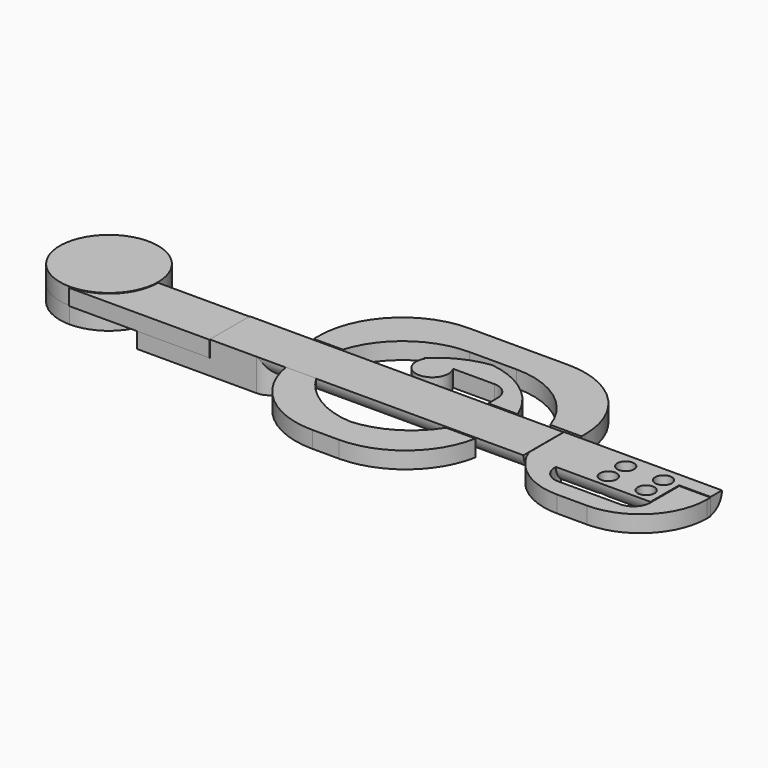
from build123d import *

# Parameters (mm, degrees)
F0_W           = 74.9647691846
F0_H           = 4.8156478442
F0_W_2         = 21.8120515347
F1_DEPTH       = 7.5
F2_T1_DEPTH    = 87.4562698657
F2_T3_DEPTH    = 17.3156478442
F2_T9_DEPTH    = 87.4562698657
F2_T13_DEPTH   = 17.3156478442
F2_T21_DEPTH   = 87.4562698657
F2_T25_DEPTH   = 17.3156478442
F4_DEPTH       = 4.8
F5_DEPTH       = 5
F6_W           = 9.4357505441
F6_H           = 4.2491005734
F7_DEPTH       = 5
F8_R           = 4.99999
F9_W           = 9.3480274081
F9_H           = 5.3821951151
F9_W_2         = 9.3480348587
F9_H_2         = 4.8156473786
F9_H_3         = 5.5238311179
F9_W_3         = 28.6106020212
F10_DEPTH      = 5
F11_T1_DEPTH   = 98.1931302685
F11_T3_DEPTH   = 105
F13_D          = 5
F14_D          = 5
F15_D          = 5
F16_D          = 5
F17_W          = 9.3480274081
F17_H          = 16.9964022934
F17_W_2        = 61.7535989732
F17_H_2        = 9.3480236828
F18_DEPTH      = 5
F17_W_3        = 9.0647486504
F17_H_3        = 12.1807572432
F17_H_4        = 8.7814740837
F17_W_4        = 39.374999702
F17_W_5        = 8.7814815342
F17_H_5        = 11.6142109036
F17_H_6        = 8.5145081393
F17_W_6        = 26.0611474514
F17_H_7        = 7.3767574504
F19_T1_DEPTH   = 5
F19_T3_DEPTH   = 5
F19_T5_DEPTH   = 130
F19_T7_DEPTH   = 130
F19_2_T1_DEPTH = 5
F19_2_T3_DEPTH = 127.8617396979
F19_2_T5_DEPTH = 128.3588691726
F19_3_T1_DEPTH = 121.4077915609
F19_3_T3_DEPTH = 93.6596472526
F20_R          = 4.8994331179
F21_DEPTH      = 5
F22_R          = 5
F22_2_R        = 5


# Not quite as in the source:
# - a fillet or chamfer that OpenCascade refuses, or shapes differently, is made with other operations: its cross-section is extruded or revolved along the edge and cut away or added
# - a fillet or chamfer is up to 0.001 mm smaller than in the source, because OpenCascade refuses the exact size


with BuildPart() as f1:
    # F0 (on Front) → F1 (new body, symmetric)
    with BuildSketch(Plane.XZ):
        with Locations((37.4823845923, 2.4078239221)):
            Rectangle(F0_W, F0_H)
        Polygon((0, -4.8156478442), (0, 0), (0, 4.8156478442), (-19.0819986165, 4.8156478442), (-19.0819986165, 0), (-19.0819986165, -4.8156478442), align=None)
        with Locations((-29.9880243838, -2.4078239221)):
            Rectangle(F0_W_2, F0_H)
    extrude(amount=F1_DEPTH, both=True)

    # F2: fillet of radius 5 on 4 edges, made by hand

    # F2_s2 → F2_t1 (cut)
    with BuildSketch(Plane.YZ):
        with BuildLine():
            ThreePointArc((-2.5033997275, 0), (-5.9731431778, 1.3998777258), (-7.5, 4.8156478442))
            Line((-7.5, 4.8156478442), (-7.5, 0))
            Line((-7.5, 0), (-2.5033997275, 0))
        make_face()
        with BuildLine():
            ThreePointArc((2.5033997275, 0), (5.9731431778, 1.3998777258), (7.5, 4.8156478442))
            Line((7.5, 4.8156478442), (7.5, 0))
            Line((7.5, 0), (2.5033997275, 0))
        make_face()
    extrude(amount=F2_T1_DEPTH, mode=Mode.SUBTRACT)

    # F2_s4 → F2_t3 (cut)
    with BuildSketch(Plane.XY.offset(-17.3156478442)):
        with BuildLine():
            ThreePointArc((0, -2.5), (-1.4644660941, -6.0355339059), (-5, -7.5))
            Line((-5, -7.5), (0, -7.5))
            Line((0, -7.5), (0, -2.5))
        make_face()
        with BuildLine():
            ThreePointArc((0, 2.5), (-1.4644660941, 6.0355339059), (-5, 7.5))
            Line((-5, 7.5), (0, 7.5))
            Line((0, 7.5), (0, 2.5))
        make_face()
    extrude(amount=F2_T3_DEPTH, mode=Mode.SUBTRACT)


with BuildPart() as f2_tool7:
    # F2_s8 → F2_t9 (new body)
    with BuildSketch(Plane.YZ.offset(-12.4915006811)):
        with BuildLine():
            ThreePointArc((-2.5033997275, 0), (-5.9731431778, 1.3998777258), (-7.5, 4.8156478442))
            Line((-7.5, 4.8156478442), (-7.5, 0))
            Line((-7.5, 0), (-2.5033997275, 0))
        make_face()
    extrude(amount=F2_T9_DEPTH)

    split(bisect_by=Plane.YZ, keep=Keep.BOTTOM)


with BuildPart() as f2_tool11:
    # F2_s12 → F2_t13 (new body)
    with BuildSketch(Plane.XY.offset(-4.8156478442)):
        with BuildLine():
            ThreePointArc((0, -2.5), (-1.4644660941, -6.0355339059), (-5, -7.5))
            Line((-5, -7.5), (0, -7.5))
            Line((0, -7.5), (0, -2.5))
        make_face()
    extrude(amount=F2_T13_DEPTH)

    split(bisect_by=Plane.XY, keep=Keep.TOP)

    split(bisect_by=Plane.XY.offset(4.8156478442), keep=Keep.BOTTOM)


with BuildPart() as f2_tool7_1:
    add(f2_tool7.part)

    # F2_t16: intersect F2_tool11
    add(f2_tool11.part, mode=Mode.INTERSECT)


with BuildPart() as f1_1:
    add(f1.part)

    # F2_t5: cut F2_tool7
    add(f2_tool7_1.part, mode=Mode.SUBTRACT)


with BuildPart() as f2_tool19:
    # F2_s20 → F2_t21 (new body)
    with BuildSketch(Plane.YZ.offset(-12.4915006811)):
        with BuildLine():
            ThreePointArc((2.5033997275, 0), (5.9731431778, 1.3998777258), (7.5, 4.8156478442))
            Line((7.5, 4.8156478442), (7.5, 0))
            Line((7.5, 0), (2.5033997275, 0))
        make_face()
    extrude(amount=F2_T21_DEPTH)

    split(bisect_by=Plane.YZ, keep=Keep.BOTTOM)


with BuildPart() as f2_tool23:
    # F2_s24 → F2_t25 (new body)
    with BuildSketch(Plane.XY.offset(-4.8156478442)):
        with BuildLine():
            ThreePointArc((0, 2.5), (-1.4644660941, 6.0355339059), (-5, 7.5))
            Line((-5, 7.5), (0, 7.5))
            Line((0, 7.5), (0, 2.5))
        make_face()
    extrude(amount=F2_T25_DEPTH)

    split(bisect_by=Plane.XY, keep=Keep.TOP)

    split(bisect_by=Plane.XY.offset(4.8156478442), keep=Keep.BOTTOM)


with BuildPart() as f2_tool19_1:
    add(f2_tool19.part)

    # F2_t28: intersect F2_tool23
    add(f2_tool23.part, mode=Mode.INTERSECT)


with BuildPart() as f1_2:
    add(f1_1.part)

    # F2_t17: cut F2_tool19
    add(f2_tool19_1.part, mode=Mode.SUBTRACT)

    # F3 (on Top) → F4 (join)
    with BuildSketch(Plane.XY):
        with BuildLine():
            Line((-61.1870549619, -7.6483818702), (-18.97931844, -7.6483818702))
            Line((-18.97931844, -7.6483818702), (-18.97931844, 7.3651091661))
            Line((-18.97931844, 7.3651091661), (-46.4570610243, 7.3651091661))
            ThreePointArc((-46.4570610243, 7.3651091661), (-50.7713763618, -3.050569434), (-61.1870549619, -7.3648847715))
            Line((-61.1870549619, -7.3648847715), (-61.1870549619, -7.6483818702))
        make_face()
    extrude(amount=F4_DEPTH)

    # F3 (on Top) → F5 (join, symmetric)
    with BuildSketch(Plane.XY):
        with BuildLine():
            ThreePointArc((-46.4570610243, 7.3651091661), (-71.602733562, 17.7807877663), (-61.1870549619, -7.3648847715))
            Line((-61.1870549619, -7.3648847715), (-61.1870549619, 7.3651091661))
            Line((-61.1870549619, 7.3651091661), (-46.4570610243, 7.3651091661))
        make_face()
        with BuildLine():
            Line((-61.1870549619, 7.3651091661), (-61.1870549619, -7.3648847715))
            ThreePointArc((-61.1870549619, -7.3648847715), (-50.7713763618, -3.050569434), (-46.4570610243, 7.3651091661))
            Line((-46.4570610243, 7.3651091661), (-61.1870549619, 7.3651091661))
        make_face()
    extrude(amount=F5_DEPTH, both=True)


with BuildPart() as f7:
    # F6 (on Top) → F7 (new body)
    with BuildSketch(Plane.XY):
        Polygon((75.2632021904, 7.365108002), (75.2632021904, -7.6483818702), (113.1341084838, -7.6483818702), (113.1341084838, 3.1160074286), (113.1341084838, 7.365108002), align=None)
        with Locations((117.8519837558, 5.2405577153)):
            Rectangle(F6_W, F6_H)
    extrude(amount=F7_DEPTH)

    # F8 (radius 5 in the source; OpenCascade refuses exactly that, so slightly less here)
    f8_edges = [f7.edges().sort_by_distance(p)[0] for p in [
        (94.198655, -7.648382, 0),
        (98.916531, 7.365108, 0),
    ]]
    fillet(f8_edges, radius=F8_R)

    # F9 (on Top) → F10 (join)
    with BuildSketch(Plane.XY):
        with Locations((80.1227204502, -15.7216731459)):
            Rectangle(F9_W, F9_H)
        Polygon((75.4487067461, -13.0305755883), (84.7967341542, -13.0305755883), (84.7967341542, -5.665468052), (75.1654356718, -5.665468052), (75.1654356718, -18.4127707034), (75.4487067461, -18.4127707034), align=None)
        with Locations((118.0813536048, -15.7216731459)):
            Rectangle(F9_W_2, F9_H)
        with Locations((118.0813536048, -10.6227518991)):
            Rectangle(F9_W_2, F9_H_2)
        with Locations((118.0813536048, -5.4530126508)):
            Rectangle(F9_W_2, F9_H_3)
        with Locations((118.0813536048, 0.0708184671)):
            Rectangle(F9_W_2, F9_H_3)
        with Locations((99.1020351648, -15.7216731459)):
            Rectangle(F9_W_3, F9_H)
    extrude(amount=F10_DEPTH)

    # F11: fillet of radius 20 on 2 edges, made by hand

    # F11_s2 → F11_t1 (cut)
    with BuildSketch(Plane.XY.offset(-46.5965651343)):
        with BuildLine():
            ThreePointArc((75.1654356718, -5.665468052), (82.5136664041, -14.9211617058), (93.8040617255, -18.4127707034))
            Line((93.8040617255, -18.4127707034), (75.1654356718, -18.4127707034))
            Line((75.1654356718, -18.4127707034), (75.1654356718, -5.665468052))
        make_face()
    extrude(amount=F11_T1_DEPTH, mode=Mode.SUBTRACT)

    # F11_s4 → F11_t3 (cut)
    with BuildSketch(Plane.XY.offset(-50)):
        with BuildLine():
            ThreePointArc((102.7553710341, -18.4127707034), (116.8975066579, -12.5549063272), (122.7553710341, 1.5872292966))
            Line((122.7553710341, 1.5872292966), (122.7553710341, -18.4127707034))
            Line((122.7553710341, -18.4127707034), (102.7553710341, -18.4127707034))
        make_face()
    extrude(amount=F11_T3_DEPTH, mode=Mode.SUBTRACT)

    # F13 (through all)
    with Locations(Plane(origin=(0, 0, 0), x_dir=(1, 0, 0), z_dir=(0, 0, -1))):
        with Locations((97.3535180092, -2.832734026)):
            Hole(F13_D / 2)

    # F14 (through all)
    with Locations(Plane(origin=(0, 0, 0), x_dir=(1, 0, 0), z_dir=(0, 0, -1))):
        with Locations((97.3535180092, 3.682554001)):
            Hole(F14_D / 2)

    # F15 (through all)
    with Locations(Plane(origin=(0, 0, 0), x_dir=(1, 0, 0), z_dir=(0, 0, -1))):
        with Locations((108.684450388, -2.832734026)):
            Hole(F15_D / 2)

    # F16 (through all)
    with Locations(Plane(origin=(0, 0, 0), x_dir=(1, 0, 0), z_dir=(0, 0, -1))):
        with Locations((108.684450388, 3.682554001)):
            Hole(F16_D / 2)

    # F22
    f22_edges = [f7.edges().sort_by_distance(p)[0] for p in [
        (113.407336, -13.030576, 2.5),
        (84.796734, -13.030576, 2.5),
    ]]
    fillet(f22_edges, radius=F22_R)


with BuildPart() as f18:
    # F17 (on Top) → F18 (new body)
    with BuildSketch(Plane.XY):
        with Locations((75.1165561378, 16.7131293565)):
            Rectangle(F17_W, F17_H)
        with Locations((39.5657429472, 29.8853423446)):
            Rectangle(F17_W_2, F17_H_2)
        with Locations((75.1165561378, 29.8853423446)):
            Rectangle(F17_W, F17_H_2)
        Polygon((8.6889434606, 7.6483818702), (8.6889434606, 25.2113305032), (8.6889434606, 34.5593541861), (0, 34.5593541861), (0, 7.6483818702), align=None)
    extrude(amount=F18_DEPTH)

    # F19: fillet of radius 25 on 4 edges, made by hand

    # F19_s2 → F19_t1 (join)
    with BuildSketch(Plane.XY):
        with BuildLine():
            ThreePointArc((70.4425424337, 8.2149282098), (61.3341564874, 20.5225336023), (46.7583193358, 25.2113305032))
            Line((46.7583193358, 25.2113305032), (70.4425424337, 25.2113305032))
            Line((70.4425424337, 25.2113305032), (70.4425424337, 8.2149282098))
        make_face()
    extrude(amount=F19_T1_DEPTH)

    # F19_s4 → F19_t3 (join)
    with BuildSketch(Plane.XY):
        with BuildLine():
            ThreePointArc((32.5571287071, 25.2113305032), (17.740352475, 20.3474458706), (8.6889434606, 7.6483818702))
            Line((8.6889434606, 7.6483818702), (8.6889434606, 25.2113305032))
            Line((8.6889434606, 25.2113305032), (32.5571287071, 25.2113305032))
        make_face()
    extrude(amount=F19_T3_DEPTH)

    # F19_s6 → F19_t5 (cut)
    with BuildSketch(Plane.XY.offset(-62.5)):
        with BuildLine():
            ThreePointArc((79.7905698419, 9.5593541861), (72.4682393715, 27.2370237157), (54.7905698419, 34.5593541861))
            Line((54.7905698419, 34.5593541861), (79.7905698419, 34.5593541861))
            Line((79.7905698419, 34.5593541861), (79.7905698419, 9.5593541861))
        make_face()
    extrude(amount=F19_T5_DEPTH, mode=Mode.SUBTRACT)

    # F19_s8 → F19_t7 (cut)
    with BuildSketch(Plane.XY.offset(-62.5)):
        with BuildLine():
            ThreePointArc((0, 9.5593541861), (7.3223304703, 27.2370237157), (25, 34.5593541861))
            Line((25, 34.5593541861), (0, 34.5593541861))
            Line((0, 34.5593541861), (0, 9.5593541861))
        make_face()
    extrude(amount=F19_T7_DEPTH, mode=Mode.SUBTRACT)


with BuildPart() as f18b:
    # F17 (on Top) → F18, piece 2 (new body)
    with BuildSketch(Plane.XY):
        with Locations((8.4056706401, -13.7387604918)):
            Rectangle(F17_W_3, F17_H_3)
        with Locations((8.4056706401, -24.2198761553)):
            Rectangle(F17_W_3, F17_H_4)
        with Locations((32.6255448163, -24.2198761553)):
            Rectangle(F17_W_4, F17_H_4)
        with Locations((56.7037854344, -14.0220336616)):
            Rectangle(F17_W_5, F17_H_5)
        with Locations((56.7037854344, -24.2198761553)):
            Rectangle(F17_W_5, F17_H_4)
    extrude(amount=F18_DEPTH)

    # F19#2: fillet of radius 25 on 4 edges, made by hand

    # F19_2_s2 → F19_2_t1 (join)
    with BuildSketch(Plane.XY):
        with BuildLine():
            ThreePointArc((52.3130446672, -8.2149282098), (43.2475475071, -16.7339870632), (31.1985792402, -19.8291391134))
            Line((31.1985792402, -19.8291391134), (52.3130446672, -19.8291391134))
            Line((52.3130446672, -19.8291391134), (52.3130446672, -8.2149282098))
        make_face()
        with BuildLine():
            ThreePointArc((34.4011997926, -19.8291391134), (22.0618535563, -16.571736347), (12.9380449653, -7.6483818702))
            Line((12.9380449653, -7.6483818702), (12.9380449653, -19.8291391134))
            Line((12.9380449653, -19.8291391134), (34.4011997926, -19.8291391134))
        make_face()
    extrude(amount=F19_2_T1_DEPTH)

    # F19_2_s4 → F19_2_t3 (cut)
    with BuildSketch(Plane.XY.offset(-61.430869849)):
        with BuildLine():
            ThreePointArc((36.5221782619, -28.6106131971), (52.4892087417, -22.8473992503), (61.0945262015, -8.2149282098))
            Line((61.0945262015, -8.2149282098), (61.0945262015, -28.6106131971))
            Line((61.0945262015, -28.6106131971), (36.5221782619, -28.6106131971))
        make_face()
    extrude(amount=F19_2_T3_DEPTH, mode=Mode.SUBTRACT)

    # F19_2_s6 → F19_2_t5 (cut)
    with BuildSketch(Plane.XY.offset(-61.6794345863)):
        with BuildLine():
            ThreePointArc((3.8732963149, -7.6483818702), (12.3577945421, -22.662440102), (28.5450701494, -28.6106131971))
            Line((28.5450701494, -28.6106131971), (3.8732963149, -28.6106131971))
            Line((3.8732963149, -28.6106131971), (3.8732963149, -7.6483818702))
        make_face()
    extrude(amount=F19_2_T5_DEPTH, mode=Mode.SUBTRACT)


with BuildPart() as f18c:
    # F17 (on Top) → F18, piece 3 (new body)
    with BuildSketch(Plane.XY):
        with Locations((56.7037854344, 11.9056359399)):
            Rectangle(F17_W_5, F17_H_6)
        with Locations((39.2824709415, 19.8512687348)):
            Rectangle(F17_W_6, F17_H_7)
        with Locations((56.7037854344, 19.8512687348)):
            Rectangle(F17_W_5, F17_H_7)
    extrude(amount=F18_DEPTH)

    # F19#3: fillet of radius 25 on 2 edges, made by hand

    # F19_3_s2 → F19_3_t1 (cut)
    with BuildSketch(Plane.XY.offset(-58.2038957804)):
        with BuildLine():
            ThreePointArc((61.0945262015, 7.6483818702), (51.9069673171, 19.1881142343), (37.8129678893, 23.53964746))
            Line((37.8129678893, 23.53964746), (61.0945262015, 23.53964746))
            Line((61.0945262015, 23.53964746), (61.0945262015, 7.6483818702))
        make_face()
    extrude(amount=F19_3_T1_DEPTH, mode=Mode.SUBTRACT)

    # F19_3_s4 → F19_3_t3 (cut)
    with BuildSketch(Plane.XY.offset(-44.3298236263)):
        with BuildLine():
            ThreePointArc((43.9838266664, 23.53964746), (34.3812505469, 21.6219032395), (26.2518972158, 16.1628900096))
            Line((26.2518972158, 16.1628900096), (26.2518972158, 23.53964746))
            Line((26.2518972158, 23.53964746), (43.9838266664, 23.53964746))
        make_face()
    extrude(amount=F19_3_T3_DEPTH, mode=Mode.SUBTRACT)

    # F20 (on Top) → F21 (join)
    with BuildSketch(Plane.XY):
        with Locations((30.7842679322, 13.5714998469)):
            Circle(F20_R)
    extrude(amount=F21_DEPTH)

    # F22#2
    f22_2_edges = [f18c.edges().sort_by_distance(p)[0] for p in [
        (52.313045, 16.16289, 2.5),
    ]]
    fillet(f22_2_edges, radius=F22_2_R)


solid = Compound([f1_2.part, f7.part, f18.part, f18b.part, f18c.part])
